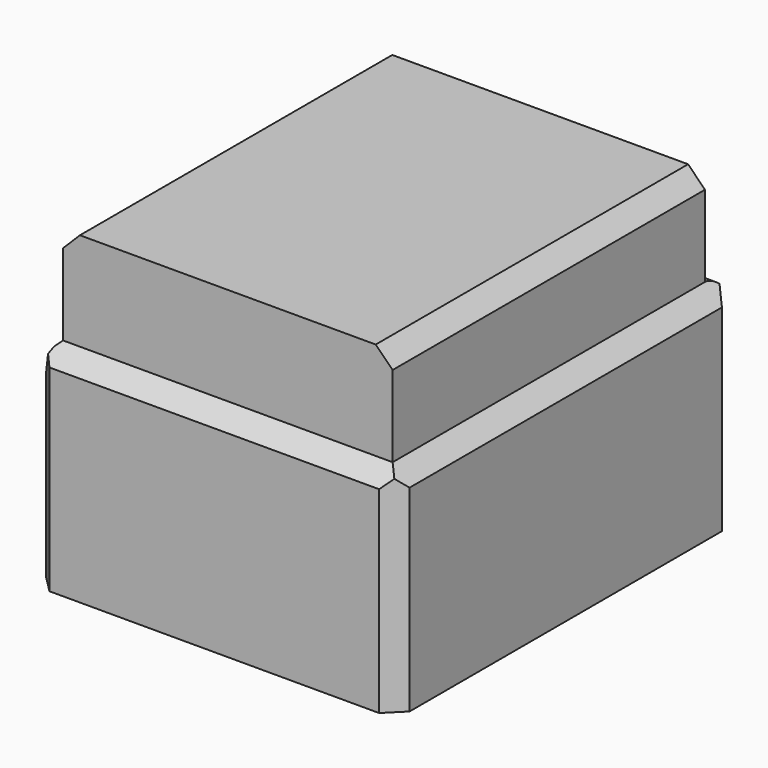
from build123d import *

# Parameters (mm, degrees)
F0_W         = 109.1705858707
F0_H         = 127.4348646402
F1_DEPTH     = 64.262
F2_SIZE      = 5.08
F3_R         = 5.08
F4_SIZE      = 5.08
F5_SIZE      = 5.08
F6_T1_DEPTH  = 85.5235311919
F7_SIZE      = 5.08
F8_SIZE      = 5.08
F9_SIZE      = 5.08
F10_DEPTH    = 29.464
F11_T1_DEPTH = 138.5363958322
F11_T3_DEPTH = 143.403163798


# Not quite as in the source:
# - a fillet or chamfer that OpenCascade refuses, or shapes differently, is made with other operations: its cross-section is extruded or revolved along the edge and cut away or added
# - two fillets or chamfers of one size are made in one step


with BuildPart() as f1:
    # F0 (on Top) → F1 (new body)
    with BuildSketch(Plane.XY):
        with Locations((2.4905838072, 0.1037716866)):
            Rectangle(F0_W, F0_H)
    extrude(amount=F1_DEPTH)

    # F2
    f2_edges = [f1.edges().sort_by_distance(p)[0] for p in [
        (57.075877, 0.103772, 64.262),
    ]]
    chamfer(f2_edges, length=F2_SIZE)

    # F3
    f3_edges = [f1.edges().sort_by_distance(p)[0] for p in [
        (-0.049416, 63.821204, 64.262),
    ]]
    fillet(f3_edges, radius=F3_R)

    # F4
    f4_edges = [f1.edges().sort_by_distance(p)[0] for p in [
        (-0.049416, -63.613661, 64.262),
    ]]
    chamfer(f4_edges, length=F4_SIZE)

    # F5
    f5_edges = [f1.edges().sort_by_distance(p)[0] for p in [
        (-52.094709, 0.103772, 64.262),
    ]]
    chamfer(f5_edges, length=F5_SIZE)

    # F6: chamfer of 5.08 on 1 edges, made by hand

    # F6_s2 → F6_t1 (cut)
    with BuildSketch(Plane.XY.offset(-13.170765596)):
        Polygon((-52.0947091281, 53.6612040067), (-48.5026066797, 62.3333064551), (-52.0947091281, 58.7412040067), align=None)
    extrude(amount=F6_T1_DEPTH, mode=Mode.SUBTRACT)

    # F7
    f7_edges = [f1.edges().sort_by_distance(p)[0] for p in [
        (-52.094709, -63.613661, 29.591),
    ]]
    chamfer(f7_edges, length=F7_SIZE)

    # F8
    f8_edges = [f1.edges().sort_by_distance(p)[0] for p in [
        (57.075877, -63.613661, 29.591),
    ]]
    chamfer(f8_edges, length=F8_SIZE)

    # F9
    f9_edges = [f1.edges().sort_by_distance(p)[0] for p in [
        (57.075877, 63.821204, 29.591),
    ]]
    chamfer(f9_edges, length=F9_SIZE)

    # F10 (add): a face of the model
    f10_faces = [f1.faces().sort_by_distance(p)[0] for p in [
        (2.4905838072, 0.1037716866, 64.262),
    ]]
    extrude(f10_faces, amount=F10_DEPTH)

    # F11: chamfer of 5.08 on 3 edges, made by hand

    # F11_s2 → F11_t1 (cut)
    with BuildSketch(Plane.XZ.offset(-66.8319696027)):
        Polygon((-52.0947091281, 54.102), (-48.5026066797, 62.7741024484), (-52.0947091281, 59.182), align=None)
    extrude(amount=F11_T1_DEPTH, mode=Mode.SUBTRACT)

    # F11_s4 → F11_t3 (cut)
    with BuildSketch(Plane.XZ.offset(-71.8053535855)):
        Polygon((51.9958767426, 88.646), (46.9158767426, 93.726), (51.9958767426, 93.726), align=None)
        Polygon((-47.0147091281, 88.646), (-41.9347091281, 93.726), (-47.0147091281, 93.726), align=None)
    extrude(amount=F11_T3_DEPTH, mode=Mode.SUBTRACT)


solid = f1.part
